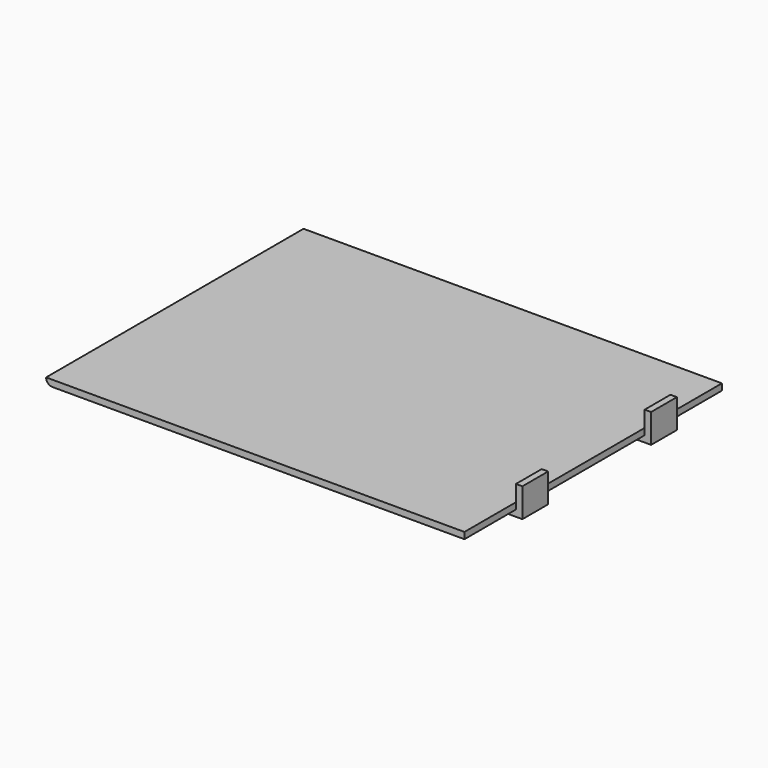
from build123d import *

# Parameters (mm, degrees)
F0_W     = 330.2
F0_H     = 5.08
F1_DEPTH = 50.8
F3_DEPTH = 25.4
F5_DEPTH = 101.6
F7_DEPTH = 25.4
F9_DEPTH = 50.8
F10_R    = 5.07999


# Not quite as in the source:
# - a fillet or chamfer is up to 0.001 mm smaller than in the source, because OpenCascade refuses the exact size


with BuildPart() as f1:
    # F0 (on Front) → F1 (new body)
    with BuildSketch(Plane.XZ):
        with Locations((5.0749575138, -2.54)):
            Rectangle(F0_W, F0_H)
    extrude(amount=F1_DEPTH)

    # F2 (on face) → F3 (join)
    with BuildSketch(Plane.XZ.offset(50.8)):
        Polygon((170.1749575138, -5.08), (170.1749575138, 0), (-160.0250424862, 0), (-160.0250424862, -5.08), (154.9349575138, -5.08), align=None)
        Polygon((170.1749575138, 12.7), (170.1749575138, 0), (170.1749575138, -5.08), (154.9349575138, -5.08), (154.9349575138, -10.16), (175.2549575138, -10.16), (175.2549575138, 12.7), align=None)
    extrude(amount=F3_DEPTH)

    # F4 (on face) → F5 (join)
    with BuildSketch(Plane.XZ.offset(76.2)):
        Polygon((170.1749575138, 0), (-160.0250424862, 0), (-160.0250424862, -5.08), (154.9349575138, -5.08), (170.1749575138, -5.08), align=None)
    extrude(amount=F5_DEPTH)

    # F6 (on face) → F7 (join)
    with BuildSketch(Plane.XZ.offset(177.8)):
        Polygon((170.1749575138, -5.08), (170.1749575138, 0), (-160.0250424862, 0), (-160.0250424862, -5.08), (154.9349575138, -5.08), align=None)
        Polygon((170.1749575138, 12.7), (170.1749575138, 0), (170.1749575138, -5.08), (154.9349575138, -5.08), (154.9349575138, -10.16), (175.2549575138, -10.16), (175.2549575138, 12.7), align=None)
    extrude(amount=F7_DEPTH)

    # F8 (on face) → F9 (join)
    with BuildSketch(Plane.XZ.offset(203.2)):
        Polygon((170.1749575138, 0), (-160.0250424862, 0), (-160.0250424862, -5.08), (154.9349575138, -5.08), (170.1749575138, -5.08), align=None)
    extrude(amount=F9_DEPTH)

    # F10 (radius 5.08 in the source; OpenCascade refuses exactly that, so slightly less here)
    f10_edges = [f1.edges().sort_by_distance(p)[0] for p in [
        (-160.025042, -127, -5.08),
    ]]
    fillet(f10_edges, radius=F10_R)


solid = f1.part
